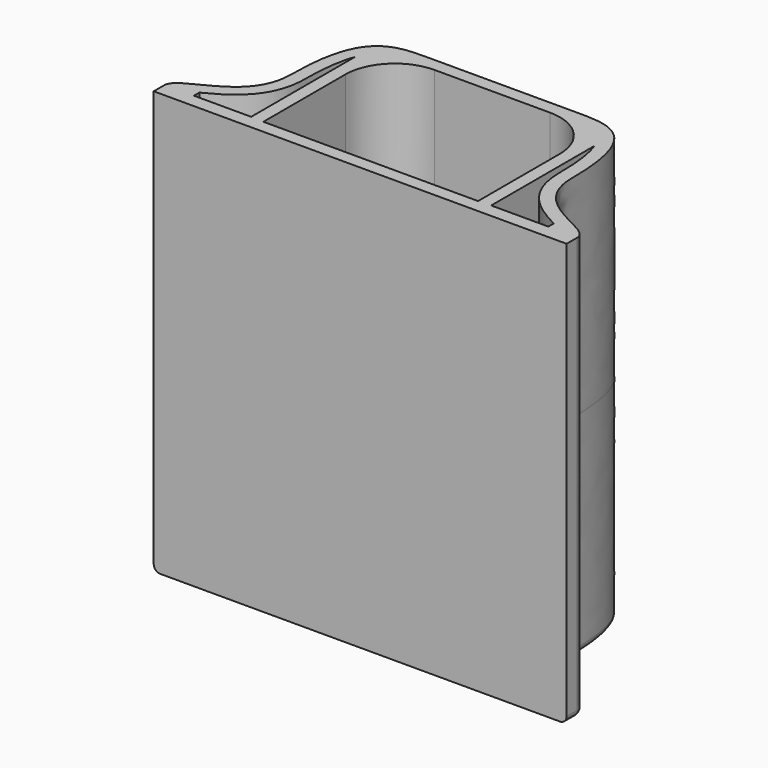
from build123d import *

# Parameters (mm, degrees)
F1_DEPTH = 32
F2_W     = 32.5
F2_H     = 23
F3_DEPTH = 61
F4_R     = 7.5
F5_R     = 2
F6_R     = 1


# Not quite as in the source:
# - ends of sketch curves that miss each other by under 0.0002 mm in the source are joined
# - the dataset's text gives a spline's control points without its knots; the knots are read off the source's solid


with BuildPart() as f1:
    # F0 (on Top) → F1 (new body, symmetric)
    with BuildSketch(Plane.XY):
        with BuildLine():
            Line((-21.25, -13.5), (21.25, -13.5))
            Line((21.25, -13.5), (31.25, -13.5))
            Line((31.25, -13.5), (31.25, -11.5198408753))
            add(Edge.make_bspline(
                [(21.25, 0), (21.25, -8.5), (31.25, -8.5), (31.25, -11.5198408753)],
                knots=[0, 0, 0, 0, 15.2547282438, 15.2547282438, 15.2547282438, 15.2547282438], degree=3))
            add(Edge.make_bspline(
                [(21.25, 0), (21.25, 13.5), (16.25, 13.5), (11.25, 13.5)],
                knots=[0, 0, 0, 0, 16.8002976164, 16.8002976164, 16.8002976164, 16.8002976164], degree=3))
            Line((11.25, 13.5), (-11.25, 13.5))
            add(Edge.make_bspline(
                [(-21.25, 0), (-21.25, 13.5), (-16.25, 13.5), (-11.25, 13.5)],
                knots=[0, 0, 0, 0, 16.8002976164, 16.8002976164, 16.8002976164, 16.8002976164], degree=3))
            add(Edge.make_bspline(
                [(-21.25, 0), (-21.25, -8.5), (-31.25, -8.5), (-31.25, -11.5198408753)],
                knots=[0, 0, 0, 0, 15.2547282438, 15.2547282438, 15.2547282438, 15.2547282438], degree=3))
            Line((-31.25, -11.5198408753), (-31.25, -13.5))
            Line((-31.25, -13.5), (-21.25, -13.5))
        make_face()
        with BuildLine():
            add(Edge.make_bspline(
                [(-19.25, 0), (-19.25, -1.1372194994), (-19.5552730118, -3.2399364358), (-20.8042939147, -5.808827997), (-22.5437726655, -7.7308676607), (-24.1392181087, -8.8909025609), (-25.3929737054, -9.6375924831), (-26.1860243265, -10.0642092729), (-26.6507400165, -10.3029893348), (-26.8250219239, -10.3918302678)],
                knots=[0, 0, 0, 0, 0.1129468247, 0.2258936493, 0.338840474, 0.4517872987, 0.508260711, 0.5647341234, 0.6002318756, 0.6002318756, 0.6002318756, 0.6002318756], degree=3))
            add(Edge.make_bspline(
                [(-19.25, 0), (-19.25, 1.6257716049), (-19.0989687266, 4.4325331187), (-18.6253639362, 6.8335979278), (-18.2732008347, 7.8796060046), (-18.167822209, 8.1526061793)],
                knots=[0, 0, 0, 0, 0.125, 0.25, 0.3001942645, 0.3001942645, 0.3001942645, 0.3001942645], degree=3))
            Line((-18.167822209, 8.1526061793), (-18.1678877172, -11.4135014336))
            Line((-18.1678877172, -11.4135014336), (-26.825022194, -11.4135014336))
            Line((-26.825022194, -11.4135014336), (-26.8250219239, -10.3918302678))
        make_face(mode=Mode.SUBTRACT)
        with BuildLine():
            Line((26.825022194, -11.4135014336), (21.25, -11.4135014336))
            Line((21.25, -11.4135014336), (18.1678877172, -11.4135014336))
            Line((18.1678877172, -11.4135014336), (18.1678877172, 8.1526314654))
            add(Edge.make_bspline(
                [(19.25, 0), (19.25, 1.6257716049), (19.0989687266, 4.4325331187), (18.6253639362, 6.8335979277), (18.2732008348, 7.8796060045), (18.1678877172, 8.1526314654)],
                knots=[0, 0, 0, 0, 0.125, 0.25, 0.3001942645, 0.3001942645, 0.3001942645, 0.3001942645], degree=3))
            add(Edge.make_bspline(
                [(19.25, 0), (19.25, -1.1372194994), (19.5552730118, -3.2399364358), (20.8042939147, -5.808827997), (22.5437726655, -7.7308676607), (24.1392181087, -8.8909025609), (25.3929737054, -9.6375924831), (26.1860243916, -10.0642093079), (26.6507401396, -10.302989398), (26.8250221032, -10.3918303593)],
                knots=[0, 0, 0, 0, 0.1129468247, 0.2258936493, 0.338840474, 0.4517872987, 0.508260711, 0.5647341234, 0.6002318877, 0.6002318877, 0.6002318877, 0.6002318877], degree=3))
            Line((26.8250221032, -10.3918303593), (26.825022194, -11.4135014336))
        make_face(mode=Mode.SUBTRACT)
    extrude(amount=F1_DEPTH, both=True)

    # F2 (on face) → F3 (cut)
    with BuildSketch(Plane.XY.offset(32)):
        Rectangle(F2_W, F2_H)
    extrude(amount=-F3_DEPTH, mode=Mode.SUBTRACT)

    # F4
    f4_edges = [f1.edges().sort_by_distance(p)[0] for p in [
        (-16.25, 11.5, 1.5),
        (16.25, 11.5, 1.5),
    ]]
    fillet(f4_edges, radius=F4_R)

    # F5
    f5_edges = [f1.edges().sort_by_distance(p)[0] for p in [
        (0, 11.5, -29),
        (-16.25, -3.75, -29),
        (-14.053301, 9.303301, -29),
        (16.25, -3.75, -29),
        (14.053301, 9.303301, -29),
    ]]
    fillet(f5_edges, radius=F5_R)

    # F6
    f6_edges = [f1.edges().sort_by_distance(p)[0] for p in [
        (0, 13.5, -32),
        (31.25, -12.50992, -32),
        (-31.25, -12.50992, -32),
        (26.25, -7.81498, -32),
        (18.125, 11.8125, -32),
        (-18.125, 11.8125, -32),
        (-26.25, -7.81498, -32),
    ]]
    fillet(f6_edges, radius=F6_R)


solid = f1.part
